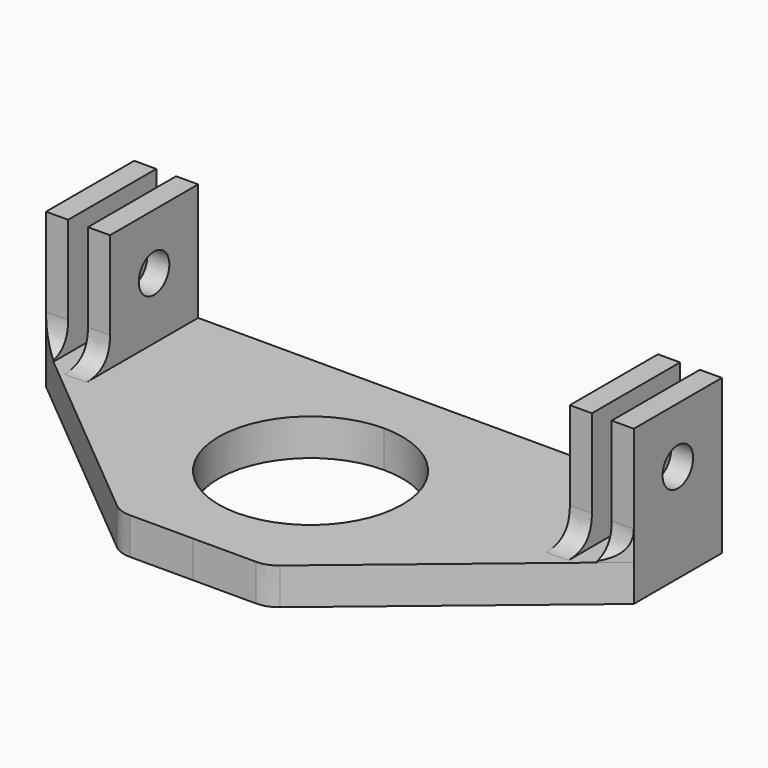
from build123d import *

# Parameters (mm, degrees)
F0_W         = 3
F0_H         = 15
F1_DEPTH     = 5
F2_DEPTH     = 16
F3_T1_DEPTH  = 3
F3_T6_DEPTH  = 23
F3_T12_DEPTH = 13
F3_T17_DEPTH = 23
F3_T20_DEPTH = 12.2409987036
F4_R         = 2.6
F5_DEPTH     = 40.0010001


# Not quite as in the source:
# - a fillet or chamfer that OpenCascade refuses, or shapes differently, is made with other operations: its cross-section is extruded or revolved along the edge and cut away or added


with BuildPart() as f1:
    # F0 (on Top) → F1 (new body)
    with BuildSketch(Plane.XY):
        with BuildLine():
            Line((-34.3, 0), (-37, 0))
            Line((-37, 0), (-37, -15))
            Line((-37, -15), (-40, -15))
            Line((-40, -15), (-10, -40))
            Line((-10, -40), (0, -40))
            Line((0, -40), (0, -32.5))
            ThreePointArc((0, -32.5), (-12.5, -20), (0, -7.5))
            Line((0, -7.5), (0, 0))
            Line((0, 0), (-31.3, 0))
            Line((-31.3, 0), (-31.3, -15))
            Line((-31.3, -15), (-34.3, -15))
            Line((-34.3, -15), (-34.3, 0))
        make_face()
        with Locations((-32.8, -7.5)):
            Rectangle(F0_W, F0_H)
        with Locations((-38.5, -7.5)):
            Rectangle(F0_W, F0_H)
    extrude(amount=-F1_DEPTH)

    # F0 (on Top) → F2 (join)
    with BuildSketch(Plane.XY):
        with Locations((-32.8, -7.5)):
            Rectangle(F0_W, F0_H)
        with Locations((-38.5, -7.5)):
            Rectangle(F0_W, F0_H)
    extrude(amount=F2_DEPTH)

    # F3: fillet of radius 4 on 3 edges, made by hand

    # F3_s2 → F3_t1 (join)
    with BuildSketch(Plane.YZ.offset(-34.3)):
        with BuildLine():
            add(Edge.make_bspline(
                [(-15, 4), (-15, 0), (-19, 0)],
                knots=[0, 0, 0, 1, 1, 1], degree=2, weights=[1, 1, 1]))
            Line((-19, 0), (-15, 0))
            Line((-15, 0), (-15, 4))
        make_face()
    extrude(amount=F3_T1_DEPTH)


with BuildPart() as f3_tool4:
    # F3_s5 → F3_t6 (new body)
    with BuildSketch(Plane.YZ.offset(-44.3)):
        with BuildLine():
            add(Edge.make_bspline(
                [(-15, 4), (-15, 0), (-19, 0)],
                knots=[0, 0, 0, 1, 1, 1], degree=2, weights=[1, 1, 1]))
            Line((-19, 0), (-15, 0))
            Line((-15, 0), (-15, 4))
        make_face()
    extrude(amount=F3_T6_DEPTH)

    split(bisect_by=Plane(origin=(-23.7704918033, -28.5245901639, 0), x_dir=(0, 0, 1), z_dir=(0.6401843997, 0.7682212796, 0)), keep=Keep.TOP)

    split(bisect_by=Plane.YZ.offset(-37), keep=Keep.BOTTOM)


with BuildPart() as f1_1:
    add(f1.part)

    # F3_t3: union F3_tool4
    add(f3_tool4.part)


with BuildPart() as f3_tool10:
    # F3_s11 → F3_t12 (new body)
    with BuildSketch(Plane.YZ.offset(-50)):
        with BuildLine():
            add(Edge.make_bspline(
                [(-15, 4), (-15, 0), (-19, 0)],
                knots=[0, 0, 0, 1, 1, 1], degree=2, weights=[1, 1, 1]))
            Line((-19, 0), (-15, 0))
            Line((-15, 0), (-15, 4))
        make_face()
    extrude(amount=F3_T12_DEPTH)

    split(bisect_by=Plane(origin=(-23.7704918033, -28.5245901639, 0), x_dir=(0, 0, 1), z_dir=(0.6401843997, 0.7682212796, 0)), keep=Keep.TOP)


with BuildPart() as f1_2:
    add(f1_1.part)

    # F3_t9: union F3_tool10
    add(f3_tool10.part)


with BuildPart() as f3_tool15:
    # F3_s16 → F3_t17 (new body)
    with BuildSketch(Plane.YZ.offset(-50)):
        with BuildLine():
            add(Edge.make_bspline(
                [(-15, 4), (-15, 0), (-19, 0)],
                knots=[0, 0, 0, 1, 1, 1], degree=2, weights=[1, 1, 1]))
            Line((-19, 0), (-15, 0))
            Line((-15, 0), (-15, 4))
        make_face()
    extrude(amount=F3_T17_DEPTH)

    split(bisect_by=Plane.YZ.offset(-31.3), keep=Keep.BOTTOM)

    split(bisect_by=Plane.YZ.offset(-34.3), keep=Keep.TOP)


with BuildPart() as f1_3:
    add(f1_2.part)

    # F3_t14: union F3_tool15
    add(f3_tool15.part)

    # F3_s21 → F3_t20 (cut)
    with BuildSketch(Plane.XY.offset(-8.6204993518)):
        with BuildLine():
            add(Edge.make_bspline(
                [(-11.1125378579, -39.0728851184), (-10, -40), (-8.5518002593, -40)],
                knots=[0, 0, 0, 1, 1, 1], degree=2, weights=[1, 1, 1]))
            Line((-8.5518002593, -40), (-10, -40))
            Line((-10, -40), (-11.1125378579, -39.0728851184))
        make_face()
    extrude(amount=F3_T20_DEPTH, mode=Mode.SUBTRACT)

    # F4 (on face) → F5 (cut, through all)
    with BuildSketch(Plane(origin=(-40, 0, 0), x_dir=(0, -1, 0), z_dir=(-1, 0, 0))):
        with Locations((7.5, 8.4)):
            Circle(F4_R)
    extrude(amount=-F5_DEPTH, mode=Mode.SUBTRACT)

    # F6: F1 across plane


with BuildPart() as f1_4:
    add(f1_3.part)
    add(f1_3.part.mirror(Plane.YZ))


solid = f1_4.part
